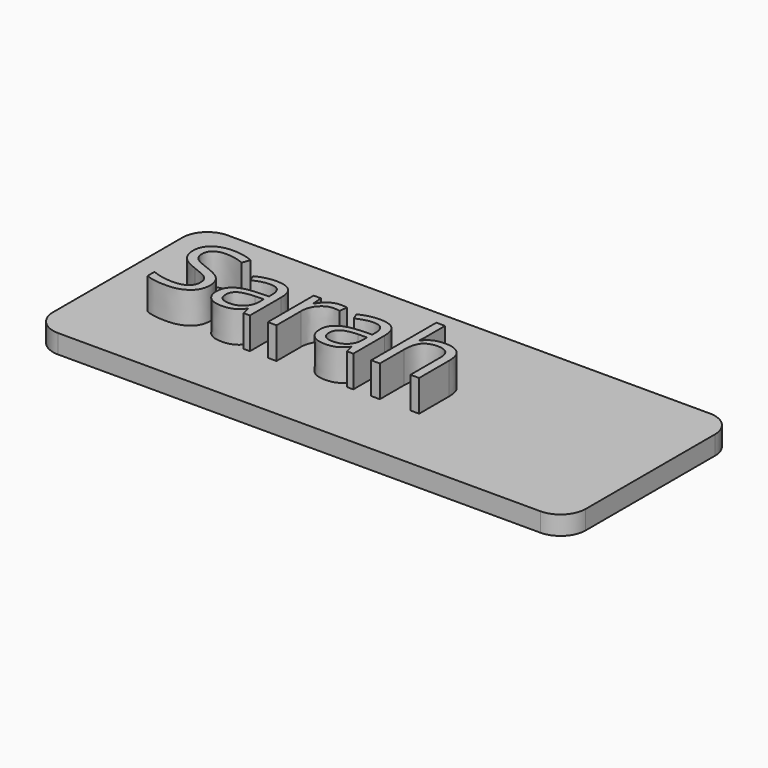
from build123d import *

# Parameters (mm, degrees)
F0_W         = 107.4794493616
F0_H         = 42.7385331132
F1_DEPTH     = 3.81
F2_R         = 5.08
F3_R         = 5.08
F4_R         = 5.08
F5_R         = 5.08
F6_TEXT_SIZE = 21.6312046784
F7_DEPTH     = 6.35


# Not quite as in the source:
# - Text() gives the source's letters only with a copy of the font that has no kerning and outlines rounded to 1/6400 em; it was checked with that copy


with BuildPart() as f1:
    # F0 (on Top) → F1 (new body)
    with BuildSketch(Plane.XY):
        with Locations((3.8075502962, -14.2099715304)):
            Rectangle(F0_W, F0_H)
    extrude(amount=F1_DEPTH)

    # F2
    f2_edges = [f1.edges().sort_by_distance(p)[0] for p in [
        (57.547275, -35.579238, 1.905),
    ]]
    fillet(f2_edges, radius=F2_R)

    # F3
    f3_edges = [f1.edges().sort_by_distance(p)[0] for p in [
        (57.547275, 7.159295, 1.905),
    ]]
    fillet(f3_edges, radius=F3_R)

    # F4
    f4_edges = [f1.edges().sort_by_distance(p)[0] for p in [
        (-49.932174, 7.159295, 1.905),
    ]]
    fillet(f4_edges, radius=F4_R)

    # F5
    f5_edges = [f1.edges().sort_by_distance(p)[0] for p in [
        (-49.932174, -35.579238, 1.905),
    ]]
    fillet(f5_edges, radius=F5_R)

    # F6 (on face) → F7 (join)
    with BuildSketch(Plane.XY.offset(3.81)):
        with Locations((-39.5469292998, -21.5294100344)):
            Text('Sarah', F6_TEXT_SIZE, font='Open Sans', text_align=(TextAlign.LEFT, TextAlign.BOTTOM))
    extrude(amount=F7_DEPTH)


solid = f1.part
